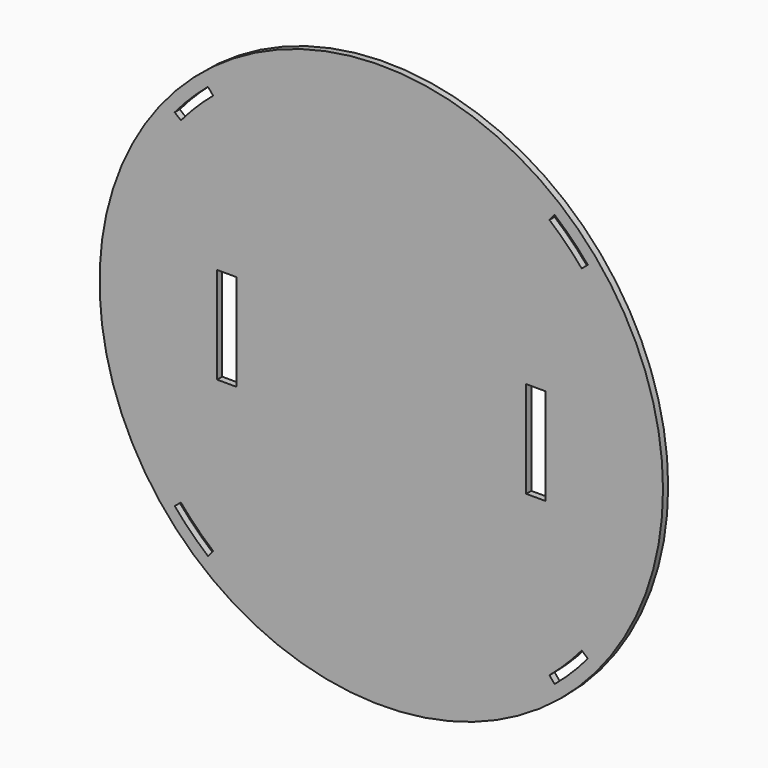
from build123d import *

# Parameters (mm, degrees)
F0_R     = 87.5
F1_DEPTH = 2


# Not quite as in the source:
# - a feature of the source that left no trace in its solid (it failed there, or was rolled back) is left out


with BuildPart() as f1:
    # F0 (on Front) → F1 (new body)
    with BuildSketch(Plane.XZ):
        Circle(F0_R)
        with BuildLine():
            ThreePointArc((-53.8334623112, -64.1562221112), (-59.2201929244, -59.2201929244), (-64.1562221112, -53.8334623112))
            Line((-64.1562221112, -53.8334623112), (-62.2411110034, -52.226493287))
            ThreePointArc((-62.2411110034, -52.226493287), (-57.4524259714, -57.4524259714), (-52.226493287, -62.2411110034))
            Line((-52.226493287, -62.2411110034), (-53.8334623112, -64.1562221112))
        make_face(mode=Mode.SUBTRACT)
        with BuildLine():
            Line((53.8334623112, -64.1562221112), (52.226493287, -62.2411110034))
            ThreePointArc((52.226493287, -62.2411110034), (57.4524259714, -57.4524259714), (62.2411110034, -52.226493287))
            Line((62.2411110034, -52.226493287), (64.1562221112, -53.8334623112))
            ThreePointArc((64.1562221112, -53.8334623112), (59.2201929244, -59.2201929244), (53.8334623112, -64.1562221112))
        make_face(mode=Mode.SUBTRACT)
        Polygon((-45, 15), (-45, 0), (-45, -15), (-51, -15), (-51, 15), align=None, mode=Mode.SUBTRACT)
        with BuildLine():
            ThreePointArc((-64.1562221112, 53.8334623112), (-59.2201929244, 59.2201929244), (-53.8334623112, 64.1562221112))
            Line((-53.8334623112, 64.1562221112), (-52.226493287, 62.2411110034))
            ThreePointArc((-52.226493287, 62.2411110034), (-57.4524259714, 57.4524259714), (-62.2411110034, 52.226493287))
            Line((-62.2411110034, 52.226493287), (-64.1562221112, 53.8334623112))
        make_face(mode=Mode.SUBTRACT)
        Polygon((51, 15), (51, -15), (45, -15), (45, 0), (45, 15), align=None, mode=Mode.SUBTRACT)
        with BuildLine():
            ThreePointArc((53.8334623112, 64.1562221112), (59.2201929244, 59.2201929244), (64.1562221112, 53.8334623112))
            Line((64.1562221112, 53.8334623112), (62.2411110034, 52.226493287))
            ThreePointArc((62.2411110034, 52.226493287), (57.4524259714, 57.4524259714), (52.226493287, 62.2411110034))
            Line((52.226493287, 62.2411110034), (53.8334623112, 64.1562221112))
        make_face(mode=Mode.SUBTRACT)
    extrude(amount=-F1_DEPTH)


solid = f1.part
